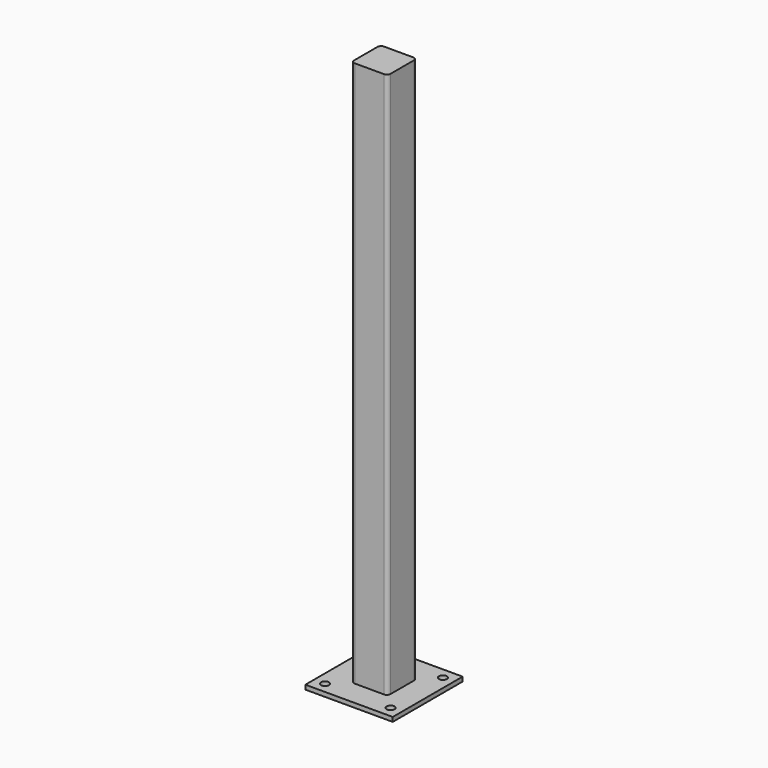
from build123d import *

# Parameters (mm, degrees)
F0_W     = 120
F0_H     = 120
F0_R     = 5.5
F1_DEPTH = 6
F2_W     = 50
F2_H     = 50
F3_DEPTH = 750
F4_R     = 5


# Not quite as in the source:
# - a feature names something its author has since deleted; it is built from what else it names


with BuildPart() as f1:
    # F0 (on Top) → F1 (new body)
    with BuildSketch(Plane.XY):
        Rectangle(F0_W, F0_H)
        with Locations((-45, -45)):
            Circle(F0_R, mode=Mode.SUBTRACT)
        with Locations((45, -45)):
            Circle(F0_R, mode=Mode.SUBTRACT)
        with Locations((-45, 45)):
            Circle(F0_R, mode=Mode.SUBTRACT)
        with Locations((45, 45)):
            Circle(F0_R, mode=Mode.SUBTRACT)
    extrude(amount=F1_DEPTH)

    # F2 (on face) → F3 (join)
    with BuildSketch(Plane.XY.offset(6)):
        Rectangle(F2_W, F2_H)
    extrude(amount=F3_DEPTH)

    # F4
    f4_edges = [f1.edges().sort_by_distance(p)[0] for p in [
        (-25, -25, 381),
        (25, -25, 381),
        (25, 25, 381),
        (-25, 25, 381),
    ]]
    fillet(f4_edges, radius=F4_R)


solid = f1.part
